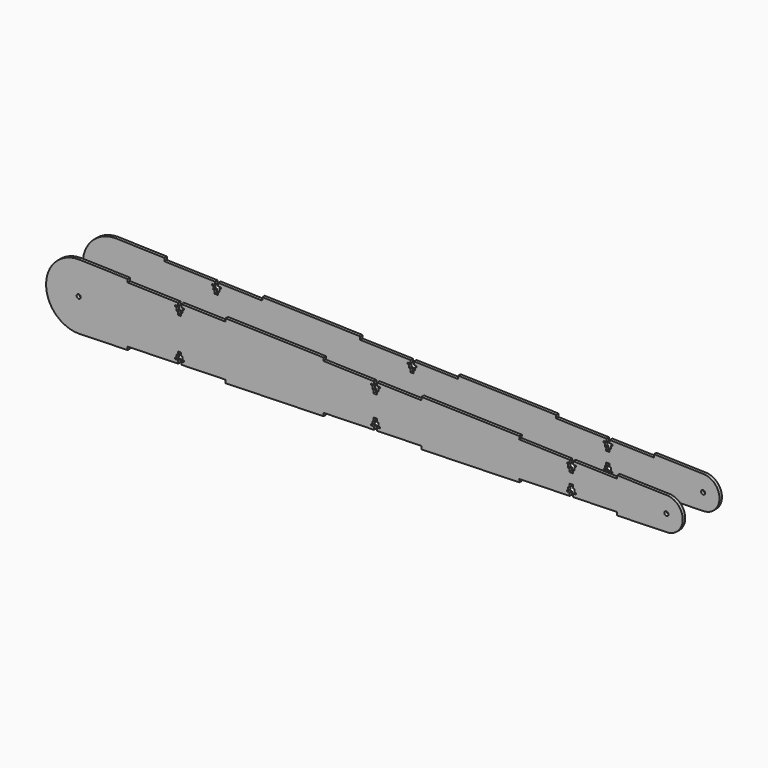
from build123d import *

# Parameters (mm, degrees)
F4_R     = 3.175
F5_DEPTH = 4.7752
F6_R     = 3.175
F7_DEPTH = 4.7752


# Not quite as in the source:
# - a variable given as a bare number and used for a length is read in inches; the dataset says mm whatever the document's units were


with BuildPart() as f5:
    # F4 (on offset) → F5 (new body)
    with BuildSketch(Plane.XZ.offset(38.1)):
        with BuildLine():
            Line((76.0380255543, 43.9107906948), (76.1706188537, 48.6841494763))
            Line((76.1706188537, 48.6841494763), (0, 50.8))
            ThreePointArc((0, 50.8), (-50.8, 0), (0, -50.8))
            Line((0, -50.8), (76.1706188537, -48.6841494763))
            Line((76.1706188537, -48.6841494763), (76.0380255543, -43.9107906948))
            Line((76.0380255543, -43.9107906948), (154.6701352089, -41.7265654266))
            Line((154.6701352089, -41.7265654266), (154.5375419094, -36.9532066451))
            Line((154.5375419094, -36.9532066451), (150.1069509127, -37.0762786172))
            Line((150.1069509127, -37.0762786172), (150.0505282321, -35.0450621145))
            Line((150.0505282321, -35.0450621145), (152.272171282, -34.9833498075))
            Line((152.272171282, -34.9833498075), (152.1311145804, -29.9053085506))
            Line((152.1311145804, -29.9053085506), (154.3400625272, -29.8439488854))
            Line((154.3400625272, -29.8439488854), (154.2032375266, -24.9182488662))
            Line((154.2032375266, -24.9182488662), (156.7549532582, -24.8473678737))
            Line((156.7549532582, -24.8473678737), (159.3066689898, -24.7764868811))
            Line((159.3066689898, -24.7764868811), (159.4434939904, -29.7021869003))
            Line((159.4434939904, -29.7021869003), (161.6524419371, -29.6408272351))
            Line((161.6524419371, -29.6408272351), (161.7934986387, -34.7188684921))
            Line((161.7934986387, -34.7188684921), (164.0151416886, -34.6571561851))
            Line((164.0151416886, -34.6571561851), (164.0715643693, -36.6883726879))
            Line((164.0715643693, -36.6883726879), (159.6409733726, -36.81144466))
            Line((159.6409733726, -36.81144466), (159.7735666721, -41.5848034415))
            Line((159.7735666721, -41.5848034415), (228.3792632617, -39.6790896474))
            Line((228.3792632617, -39.6790896474), (228.5118565612, -44.4524484289))
            Line((228.5118565612, -44.4524484289), (380.8530942687, -40.2207473814))
            Line((380.8530942687, -40.2207473814), (380.7205009692, -35.4473885999))
            Line((380.7205009692, -35.4473885999), (459.3526106238, -33.2631633317))
            Line((459.3526106238, -33.2631633317), (459.2200173243, -28.4898045502))
            Line((459.2200173243, -28.4898045502), (454.7894263277, -28.6128765224))
            Line((454.7894263277, -28.6128765224), (454.7330036471, -26.5816600196))
            Line((454.7330036471, -26.5816600196), (456.954646697, -26.5199477127))
            Line((456.954646697, -26.5199477127), (456.8135899954, -21.4419064557))
            Line((456.8135899954, -21.4419064557), (459.0225379421, -21.3805467906))
            Line((459.0225379421, -21.3805467906), (458.8857129416, -16.4548467714))
            Line((458.8857129416, -16.4548467714), (461.4374286732, -16.3839657788))
            Line((461.4374286732, -16.3839657788), (463.9891444048, -16.3130847863))
            Line((463.9891444048, -16.3130847863), (464.1259694053, -21.2387848055))
            Line((464.1259694053, -21.2387848055), (466.3349173521, -21.1774251403))
            Line((466.3349173521, -21.1774251403), (466.4759740537, -26.2554663972))
            Line((466.4759740537, -26.2554663972), (468.6976171036, -26.1937540903))
            Line((468.6976171036, -26.1937540903), (468.7540397842, -28.224970593))
            Line((468.7540397842, -28.224970593), (464.3234487875, -28.3480425652))
            Line((464.3234487875, -28.3480425652), (464.456042087, -33.1214013467))
            Line((464.456042087, -33.1214013467), (533.0617386767, -31.2156875525))
            Line((533.0617386767, -31.2156875525), (533.1943319762, -35.989046334))
            Line((533.1943319762, -35.989046334), (685.5355696836, -31.7573452866))
            Line((685.5355696836, -31.7573452866), (685.4029763841, -26.9839865051))
            Line((685.4029763841, -26.9839865051), (764.0350860388, -24.7997612369))
            Line((764.0350860388, -24.7997612369), (763.9024927393, -20.0264024554))
            Line((763.9024927393, -20.0264024554), (759.4719017426, -20.1494744275))
            Line((759.4719017426, -20.1494744275), (759.415479062, -18.1182579247))
            Line((759.415479062, -18.1182579247), (761.6371221119, -18.0565456178))
            Line((761.6371221119, -18.0565456178), (761.4960654103, -12.9785043609))
            Line((761.4960654103, -12.9785043609), (763.7050133571, -12.9171446957))
            Line((763.7050133571, -12.9171446957), (763.5681883565, -7.9914446765))
            Line((763.5681883565, -7.9914446765), (766.1199040881, -7.9205636839))
            Line((766.1199040881, -7.9205636839), (768.6716198197, -7.8496826914))
            Line((768.6716198197, -7.8496826914), (768.8084448203, -12.7753827106))
            Line((768.8084448203, -12.7753827106), (771.017392767, -12.7140230454))
            Line((771.017392767, -12.7140230454), (771.1584494686, -17.7920643023))
            Line((771.1584494686, -17.7920643023), (773.3800925185, -17.7303519954))
            Line((773.3800925185, -17.7303519954), (773.4365151992, -19.7615684982))
            Line((773.4365151992, -19.7615684982), (769.0059242025, -19.8846404703))
            Line((769.0059242025, -19.8846404703), (769.138517502, -24.6579992518))
            Line((769.138517502, -24.6579992518), (837.7442140916, -22.7522854576))
            Line((837.7442140916, -22.7522854576), (837.8768073911, -27.5256442391))
            Line((837.8768073911, -27.5256442391), (914.4, -25.4))
            ThreePointArc((914.4, -25.4), (939.8, 0), (914.4, 25.4))
            Line((914.4, 25.4), (837.8768073911, 27.5256442391))
            Line((837.8768073911, 27.5256442391), (837.7442140916, 22.7522854576))
            Line((837.7442140916, 22.7522854576), (769.138517502, 24.6579992518))
            Line((769.138517502, 24.6579992518), (769.0059242025, 19.8846404703))
            Line((769.0059242025, 19.8846404703), (773.4365151992, 19.7615684982))
            Line((773.4365151992, 19.7615684982), (773.3800925185, 17.7303519954))
            Line((773.3800925185, 17.7303519954), (771.1584494686, 17.7920643023))
            Line((771.1584494686, 17.7920643023), (771.017392767, 12.7140230454))
            Line((771.017392767, 12.7140230454), (768.8084448203, 12.7753827106))
            Line((768.8084448203, 12.7753827106), (768.6716198197, 7.8496826914))
            Line((768.6716198197, 7.8496826914), (766.1199040881, 7.9205636839))
            Line((766.1199040881, 7.9205636839), (763.5681883565, 7.9914446765))
            Line((763.5681883565, 7.9914446765), (763.7050133571, 12.9171446957))
            Line((763.7050133571, 12.9171446957), (761.4960654103, 12.9785043609))
            Line((761.4960654103, 12.9785043609), (761.6371221119, 18.0565456178))
            Line((761.6371221119, 18.0565456178), (759.415479062, 18.1182579247))
            Line((759.415479062, 18.1182579247), (759.4719017426, 20.1494744275))
            Line((759.4719017426, 20.1494744275), (763.9024927393, 20.0264024554))
            Line((763.9024927393, 20.0264024554), (764.0350860388, 24.7997612369))
            Line((764.0350860388, 24.7997612369), (685.4029763841, 26.9839865051))
            Line((685.4029763841, 26.9839865051), (685.5355696836, 31.7573452866))
            Line((685.5355696836, 31.7573452866), (533.1943319762, 35.989046334))
            Line((533.1943319762, 35.989046334), (533.0617386767, 31.2156875525))
            Line((533.0617386767, 31.2156875525), (464.456042087, 33.1214013467))
            Line((464.456042087, 33.1214013467), (464.3234487875, 28.3480425652))
            Line((464.3234487875, 28.3480425652), (468.7540397842, 28.224970593))
            Line((468.7540397842, 28.224970593), (468.6976171036, 26.1937540903))
            Line((468.6976171036, 26.1937540903), (466.4759740537, 26.2554663972))
            Line((466.4759740537, 26.2554663972), (466.3349173521, 21.1774251403))
            Line((466.3349173521, 21.1774251403), (464.1259694053, 21.2387848055))
            Line((464.1259694053, 21.2387848055), (463.9891444048, 16.3130847863))
            Line((463.9891444048, 16.3130847863), (461.4374286732, 16.3839657788))
            Line((461.4374286732, 16.3839657788), (458.8857129416, 16.4548467713))
            Line((458.8857129416, 16.4548467713), (459.0225379421, 21.3805467906))
            Line((459.0225379421, 21.3805467906), (456.8135899954, 21.4419064557))
            Line((456.8135899954, 21.4419064557), (456.954646697, 26.5199477127))
            Line((456.954646697, 26.5199477127), (454.7330036471, 26.5816600196))
            Line((454.7330036471, 26.5816600196), (454.7894263277, 28.6128765224))
            Line((454.7894263277, 28.6128765224), (459.2200173243, 28.4898045502))
            Line((459.2200173243, 28.4898045502), (459.3526106238, 33.2631633317))
            Line((459.3526106238, 33.2631633317), (380.7205009692, 35.4473885999))
            Line((380.7205009692, 35.4473885999), (380.8530942687, 40.2207473814))
            Line((380.8530942687, 40.2207473814), (228.5118565612, 44.4524484289))
            Line((228.5118565612, 44.4524484289), (228.3792632617, 39.6790896474))
            Line((228.3792632617, 39.6790896474), (159.7735666721, 41.5848034415))
            Line((159.7735666721, 41.5848034415), (159.6409733726, 36.81144466))
            Line((159.6409733726, 36.81144466), (164.0715643693, 36.6883726879))
            Line((164.0715643693, 36.6883726879), (164.0151416886, 34.6571561851))
            Line((164.0151416886, 34.6571561851), (161.7934986387, 34.7188684921))
            Line((161.7934986387, 34.7188684921), (161.6524419371, 29.6408272351))
            Line((161.6524419371, 29.6408272351), (159.4434939904, 29.7021869003))
            Line((159.4434939904, 29.7021869003), (159.3066689898, 24.7764868811))
            Line((159.3066689898, 24.7764868811), (156.7549532582, 24.8473678737))
            Line((156.7549532582, 24.8473678737), (154.2032375266, 24.9182488662))
            Line((154.2032375266, 24.9182488662), (154.3400625272, 29.8439488854))
            Line((154.3400625272, 29.8439488854), (152.1311145804, 29.9053085506))
            Line((152.1311145804, 29.9053085506), (152.272171282, 34.9833498075))
            Line((152.272171282, 34.9833498075), (150.0505282321, 35.0450621145))
            Line((150.0505282321, 35.0450621145), (150.1069509127, 37.0762786172))
            Line((150.1069509127, 37.0762786172), (154.5375419094, 36.9532066451))
            Line((154.5375419094, 36.9532066451), (154.6701352089, 41.7265654266))
            Line((154.6701352089, 41.7265654266), (76.0380255543, 43.9107906948))
        make_face()
        Circle(F4_R, mode=Mode.SUBTRACT)
        with Locations((914.4, 0)):
            Circle(F4_R, mode=Mode.SUBTRACT)
    extrude(amount=-F5_DEPTH)


with BuildPart() as f7:
    # F6 (on offset) → F7 (new body)
    with BuildSketch(Plane.XZ.offset(-38.1)):
        with BuildLine():
            Line((76.0380255543, 43.9107906948), (76.1706188537, 48.6841494763))
            Line((76.1706188537, 48.6841494763), (0, 50.8))
            ThreePointArc((0, 50.8), (-50.8, 0), (0, -50.8))
            Line((0, -50.8), (76.1706188537, -48.6841494763))
            Line((76.1706188537, -48.6841494763), (76.0380255543, -43.9107906948))
            Line((76.0380255543, -43.9107906948), (154.6701352089, -41.7265654266))
            Line((154.6701352089, -41.7265654266), (154.5375419094, -36.9532066451))
            Line((154.5375419094, -36.9532066451), (150.1069509127, -37.0762786172))
            Line((150.1069509127, -37.0762786172), (150.0505282321, -35.0450621145))
            Line((150.0505282321, -35.0450621145), (152.272171282, -34.9833498075))
            Line((152.272171282, -34.9833498075), (152.1311145804, -29.9053085506))
            Line((152.1311145804, -29.9053085506), (154.3400625272, -29.8439488854))
            Line((154.3400625272, -29.8439488854), (154.2032375266, -24.9182488662))
            Line((154.2032375266, -24.9182488662), (156.7549532582, -24.8473678737))
            Line((156.7549532582, -24.8473678737), (159.3066689898, -24.7764868811))
            Line((159.3066689898, -24.7764868811), (159.4434939904, -29.7021869003))
            Line((159.4434939904, -29.7021869003), (161.6524419371, -29.6408272351))
            Line((161.6524419371, -29.6408272351), (161.7934986387, -34.7188684921))
            Line((161.7934986387, -34.7188684921), (164.0151416886, -34.6571561851))
            Line((164.0151416886, -34.6571561851), (164.0715643693, -36.6883726879))
            Line((164.0715643693, -36.6883726879), (159.6409733726, -36.81144466))
            Line((159.6409733726, -36.81144466), (159.7735666721, -41.5848034415))
            Line((159.7735666721, -41.5848034415), (228.3792632617, -39.6790896474))
            Line((228.3792632617, -39.6790896474), (228.5118565612, -44.4524484289))
            Line((228.5118565612, -44.4524484289), (380.8530942687, -40.2207473814))
            Line((380.8530942687, -40.2207473814), (380.7205009692, -35.4473885999))
            Line((380.7205009692, -35.4473885999), (459.3526106238, -33.2631633317))
            Line((459.3526106238, -33.2631633317), (459.2200173243, -28.4898045502))
            Line((459.2200173243, -28.4898045502), (454.7894263277, -28.6128765224))
            Line((454.7894263277, -28.6128765224), (454.7330036471, -26.5816600196))
            Line((454.7330036471, -26.5816600196), (456.954646697, -26.5199477127))
            Line((456.954646697, -26.5199477127), (456.8135899954, -21.4419064557))
            Line((456.8135899954, -21.4419064557), (459.0225379421, -21.3805467906))
            Line((459.0225379421, -21.3805467906), (458.8857129416, -16.4548467714))
            Line((458.8857129416, -16.4548467714), (461.4374286732, -16.3839657788))
            Line((461.4374286732, -16.3839657788), (463.9891444048, -16.3130847863))
            Line((463.9891444048, -16.3130847863), (464.1259694053, -21.2387848055))
            Line((464.1259694053, -21.2387848055), (466.3349173521, -21.1774251403))
            Line((466.3349173521, -21.1774251403), (466.4759740537, -26.2554663972))
            Line((466.4759740537, -26.2554663972), (468.6976171036, -26.1937540903))
            Line((468.6976171036, -26.1937540903), (468.7540397842, -28.224970593))
            Line((468.7540397842, -28.224970593), (464.3234487875, -28.3480425652))
            Line((464.3234487875, -28.3480425652), (464.456042087, -33.1214013467))
            Line((464.456042087, -33.1214013467), (533.0617386767, -31.2156875525))
            Line((533.0617386767, -31.2156875525), (533.1943319762, -35.989046334))
            Line((533.1943319762, -35.989046334), (685.5355696836, -31.7573452866))
            Line((685.5355696836, -31.7573452866), (685.4029763841, -26.9839865051))
            Line((685.4029763841, -26.9839865051), (764.0350860388, -24.7997612369))
            Line((764.0350860388, -24.7997612369), (763.9024927393, -20.0264024554))
            Line((763.9024927393, -20.0264024554), (759.4719017426, -20.1494744275))
            Line((759.4719017426, -20.1494744275), (759.415479062, -18.1182579247))
            Line((759.415479062, -18.1182579247), (761.6371221119, -18.0565456178))
            Line((761.6371221119, -18.0565456178), (761.4960654103, -12.9785043609))
            Line((761.4960654103, -12.9785043609), (763.7050133571, -12.9171446957))
            Line((763.7050133571, -12.9171446957), (763.5681883565, -7.9914446765))
            Line((763.5681883565, -7.9914446765), (766.1199040881, -7.9205636839))
            Line((766.1199040881, -7.9205636839), (768.6716198197, -7.8496826914))
            Line((768.6716198197, -7.8496826914), (768.8084448203, -12.7753827106))
            Line((768.8084448203, -12.7753827106), (771.017392767, -12.7140230454))
            Line((771.017392767, -12.7140230454), (771.1584494686, -17.7920643023))
            Line((771.1584494686, -17.7920643023), (773.3800925185, -17.7303519954))
            Line((773.3800925185, -17.7303519954), (773.4365151992, -19.7615684982))
            Line((773.4365151992, -19.7615684982), (769.0059242025, -19.8846404703))
            Line((769.0059242025, -19.8846404703), (769.138517502, -24.6579992518))
            Line((769.138517502, -24.6579992518), (837.7442140916, -22.7522854576))
            Line((837.7442140916, -22.7522854576), (837.8768073911, -27.5256442391))
            Line((837.8768073911, -27.5256442391), (914.4, -25.4))
            ThreePointArc((914.4, -25.4), (939.8, 0), (914.4, 25.4))
            Line((914.4, 25.4), (837.8768073911, 27.5256442391))
            Line((837.8768073911, 27.5256442391), (837.7442140916, 22.7522854576))
            Line((837.7442140916, 22.7522854576), (769.138517502, 24.6579992518))
            Line((769.138517502, 24.6579992518), (769.0059242025, 19.8846404703))
            Line((769.0059242025, 19.8846404703), (773.4365151992, 19.7615684982))
            Line((773.4365151992, 19.7615684982), (773.3800925185, 17.7303519954))
            Line((773.3800925185, 17.7303519954), (771.1584494686, 17.7920643023))
            Line((771.1584494686, 17.7920643023), (771.017392767, 12.7140230454))
            Line((771.017392767, 12.7140230454), (768.8084448203, 12.7753827106))
            Line((768.8084448203, 12.7753827106), (768.6716198197, 7.8496826914))
            Line((768.6716198197, 7.8496826914), (766.1199040881, 7.9205636839))
            Line((766.1199040881, 7.9205636839), (763.5681883565, 7.9914446765))
            Line((763.5681883565, 7.9914446765), (763.7050133571, 12.9171446957))
            Line((763.7050133571, 12.9171446957), (761.4960654103, 12.9785043609))
            Line((761.4960654103, 12.9785043609), (761.6371221119, 18.0565456178))
            Line((761.6371221119, 18.0565456178), (759.415479062, 18.1182579247))
            Line((759.415479062, 18.1182579247), (759.4719017426, 20.1494744275))
            Line((759.4719017426, 20.1494744275), (763.9024927393, 20.0264024554))
            Line((763.9024927393, 20.0264024554), (764.0350860388, 24.7997612369))
            Line((764.0350860388, 24.7997612369), (685.4029763841, 26.9839865051))
            Line((685.4029763841, 26.9839865051), (685.5355696836, 31.7573452866))
            Line((685.5355696836, 31.7573452866), (533.1943319762, 35.989046334))
            Line((533.1943319762, 35.989046334), (533.0617386767, 31.2156875525))
            Line((533.0617386767, 31.2156875525), (464.456042087, 33.1214013467))
            Line((464.456042087, 33.1214013467), (464.3234487875, 28.3480425652))
            Line((464.3234487875, 28.3480425652), (468.7540397842, 28.224970593))
            Line((468.7540397842, 28.224970593), (468.6976171036, 26.1937540903))
            Line((468.6976171036, 26.1937540903), (466.4759740537, 26.2554663972))
            Line((466.4759740537, 26.2554663972), (466.3349173521, 21.1774251403))
            Line((466.3349173521, 21.1774251403), (464.1259694053, 21.2387848055))
            Line((464.1259694053, 21.2387848055), (463.9891444048, 16.3130847863))
            Line((463.9891444048, 16.3130847863), (461.4374286732, 16.3839657788))
            Line((461.4374286732, 16.3839657788), (458.8857129416, 16.4548467713))
            Line((458.8857129416, 16.4548467713), (459.0225379421, 21.3805467906))
            Line((459.0225379421, 21.3805467906), (456.8135899954, 21.4419064557))
            Line((456.8135899954, 21.4419064557), (456.954646697, 26.5199477127))
            Line((456.954646697, 26.5199477127), (454.7330036471, 26.5816600196))
            Line((454.7330036471, 26.5816600196), (454.7894263277, 28.6128765224))
            Line((454.7894263277, 28.6128765224), (459.2200173243, 28.4898045502))
            Line((459.2200173243, 28.4898045502), (459.3526106238, 33.2631633317))
            Line((459.3526106238, 33.2631633317), (380.7205009692, 35.4473885999))
            Line((380.7205009692, 35.4473885999), (380.8530942687, 40.2207473814))
            Line((380.8530942687, 40.2207473814), (228.5118565612, 44.4524484289))
            Line((228.5118565612, 44.4524484289), (228.3792632617, 39.6790896474))
            Line((228.3792632617, 39.6790896474), (159.7735666721, 41.5848034415))
            Line((159.7735666721, 41.5848034415), (159.6409733726, 36.81144466))
            Line((159.6409733726, 36.81144466), (164.0715643693, 36.6883726879))
            Line((164.0715643693, 36.6883726879), (164.0151416886, 34.6571561851))
            Line((164.0151416886, 34.6571561851), (161.7934986387, 34.7188684921))
            Line((161.7934986387, 34.7188684921), (161.6524419371, 29.6408272351))
            Line((161.6524419371, 29.6408272351), (159.4434939904, 29.7021869003))
            Line((159.4434939904, 29.7021869003), (159.3066689898, 24.7764868811))
            Line((159.3066689898, 24.7764868811), (156.7549532582, 24.8473678737))
            Line((156.7549532582, 24.8473678737), (154.2032375266, 24.9182488662))
            Line((154.2032375266, 24.9182488662), (154.3400625272, 29.8439488854))
            Line((154.3400625272, 29.8439488854), (152.1311145804, 29.9053085506))
            Line((152.1311145804, 29.9053085506), (152.272171282, 34.9833498075))
            Line((152.272171282, 34.9833498075), (150.0505282321, 35.0450621145))
            Line((150.0505282321, 35.0450621145), (150.1069509127, 37.0762786172))
            Line((150.1069509127, 37.0762786172), (154.5375419094, 36.9532066451))
            Line((154.5375419094, 36.9532066451), (154.6701352089, 41.7265654266))
            Line((154.6701352089, 41.7265654266), (76.0380255543, 43.9107906948))
        make_face()
        Circle(F6_R, mode=Mode.SUBTRACT)
        with Locations((914.4, 0)):
            Circle(F6_R, mode=Mode.SUBTRACT)
    extrude(amount=F7_DEPTH)


solid = Compound([f5.part, f7.part])
